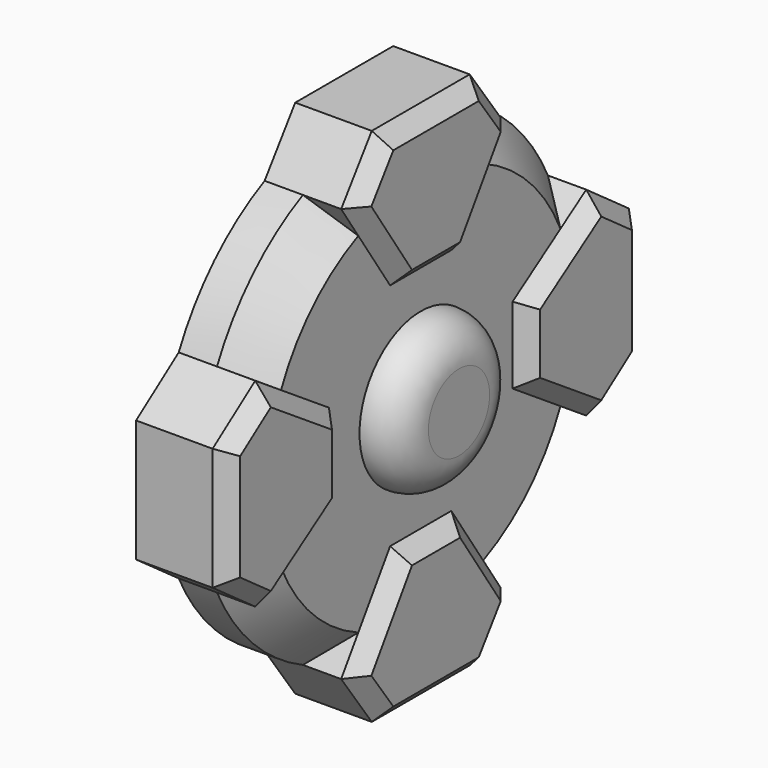
from build123d import *

# Parameters (mm, degrees)
F1_DEPTH = 10
F2_DEPTH = 12
F3_SIZE  = 5
F4_SIZE  = 1.99999
F5_R     = 10
F6_DEPTH = 5
F7_R     = 4.99999
F9_DEPTH = 9


# Not quite as in the source:
# - a fillet or chamfer is up to 0.001 mm smaller than in the source, because OpenCascade refuses the exact size


with BuildPart() as f1:
    # F0 (on Right) → F1 (new body)
    with BuildSketch(Plane.YZ):
        with BuildLine():
            Line((15, 5), (27.0370116692, 13))
            ThreePointArc((27.0370116692, 13), (21.2132034356, 21.2132034356), (13, 27.0370116692))
            Line((13, 27.0370116692), (5, 15))
            Line((5, 15), (0, 15))
            Line((0, 15), (-5, 15))
            Line((-5, 15), (-13, 27.0370116692))
            ThreePointArc((-13, 27.0370116692), (-21.2132034356, 21.2132034356), (-27.0370116692, 13))
            Line((-27.0370116692, 13), (-15, 5))
            Line((-15, 5), (-15, 0))
            Line((-15, 0), (-15, -5))
            Line((-15, -5), (-27.0370116692, -13))
            ThreePointArc((-27.0370116692, -13), (-21.2132034356, -21.2132034356), (-13, -27.0370116692))
            Line((-13, -27.0370116692), (-5, -15))
            Line((-5, -15), (0, -15))
            Line((0, -15), (5, -15))
            Line((5, -15), (13, -27.0370116692))
            ThreePointArc((13, -27.0370116692), (21.2132034356, -21.2132034356), (27.0370116692, -13))
            Line((27.0370116692, -13), (15, -5))
            Line((15, -5), (15, 0))
            Line((15, 0), (15, 5))
        make_face()
    extrude(amount=F1_DEPTH)

    # F0 (on Right) → F2 (join)
    with BuildSketch(Plane.YZ):
        with BuildLine():
            ThreePointArc((27.0370116692, -13), (29.2498747867, -6.6666952054), (30, 0))
            ThreePointArc((30, 0), (29.2498747867, 6.6666952054), (27.0370116692, 13))
            Line((27.0370116692, 13), (15, 5))
            Line((15, 5), (15, 0))
            Line((15, 0), (15, -5))
            Line((15, -5), (27.0370116692, -13))
        make_face()
        with BuildLine():
            ThreePointArc((27.0370116692, 13), (29.2498747867, 6.6666952054), (30, 0))
            ThreePointArc((30, 0), (29.2498747867, -6.6666952054), (27.0370116692, -13))
            Line((27.0370116692, -13), (34, -8))
            Line((34, -8), (34, 0))
            Line((34, 0), (34, 8))
            Line((34, 8), (27.0370116692, 13))
        make_face()
        with BuildLine():
            Line((5, 15), (13, 27.0370116692))
            ThreePointArc((13, 27.0370116692), (0, 30), (-13, 27.0370116692))
            Line((-13, 27.0370116692), (-5, 15))
            Line((-5, 15), (0, 15))
            Line((0, 15), (5, 15))
        make_face()
        with BuildLine():
            ThreePointArc((-13, 27.0370116692), (0, 30), (13, 27.0370116692))
            Line((13, 27.0370116692), (8, 34))
            Line((8, 34), (0, 34))
            Line((0, 34), (-8, 34))
            Line((-8, 34), (-13, 27.0370116692))
        make_face()
        with BuildLine():
            Line((-15, 5), (-27.0370116692, 13))
            ThreePointArc((-27.0370116692, 13), (-30, 0), (-27.0370116692, -13))
            Line((-27.0370116692, -13), (-15, -5))
            Line((-15, -5), (-15, 0))
            Line((-15, 0), (-15, 5))
        make_face()
        with BuildLine():
            ThreePointArc((-27.0370116692, -13), (-30, 0), (-27.0370116692, 13))
            Line((-27.0370116692, 13), (-34, 8))
            Line((-34, 8), (-34, 0))
            Line((-34, 0), (-34, -8))
            Line((-34, -8), (-27.0370116692, -13))
        make_face()
        with BuildLine():
            ThreePointArc((-13, -27.0370116692), (0, -30), (13, -27.0370116692))
            Line((13, -27.0370116692), (5, -15))
            Line((5, -15), (0, -15))
            Line((0, -15), (-5, -15))
            Line((-5, -15), (-13, -27.0370116692))
        make_face()
        with BuildLine():
            Line((8, -34), (13, -27.0370116692))
            ThreePointArc((13, -27.0370116692), (0, -30), (-13, -27.0370116692))
            Line((-13, -27.0370116692), (-8, -34))
            Line((-8, -34), (0, -34))
            Line((0, -34), (8, -34))
        make_face()
    extrude(amount=F2_DEPTH)

    # F3
    f3_edges = [f1.edges().sort_by_distance(p)[0] for p in [
        (10, 21.213203, 21.213203),
        (10, -21.213203, 21.213203),
        (10, -21.213203, -21.213203),
        (10, 21.213203, -21.213203),
    ]]
    chamfer(f3_edges, length=F3_SIZE)

    # F4 (size 2 in the source; OpenCascade refuses exactly that, so slightly less here)
    f4_edges = [f1.edges().sort_by_distance(p)[0] for p in [
        (12, 0, 34),
        (12, -10.5, 30.518506),
        (12, 10.5, 30.518506),
        (12, -9, 21.018506),
        (12, 9, 21.018506),
        (12, 0, 15),
        (12, -15, 0),
        (12, -21.018506, 9),
        (12, -30.518506, 10.5),
        (12, -34, 0),
        (12, -30.518506, -10.5),
        (12, -21.018506, -9),
        (12, 0, -15),
        (12, -9, -21.018506),
        (12, -10.5, -30.518506),
        (12, 0, -34),
        (12, 10.5, -30.518506),
        (12, 9, -21.018506),
        (12, 15, 0),
        (12, 21.018506, 9),
        (12, 30.518506, 10.5),
        (12, 34, 0),
        (12, 21.018506, -9),
        (12, 30.518506, -10.5),
    ]]
    chamfer(f4_edges, length=F4_SIZE)

    # F5 (on face) → F6 (join)
    with BuildSketch(Plane.YZ.offset(10)):
        Circle(F5_R)
    extrude(amount=F6_DEPTH)

    # F7 (radius 5 in the source; OpenCascade refuses exactly that, so slightly less here)
    f7_edges = [f1.edges().sort_by_distance(p)[0] for p in [
        (15, -10, 0),
    ]]
    fillet(f7_edges, radius=F7_R)

    # F8 (on face) → F9 (join)
    with BuildSketch(Plane.YZ):
        with BuildLine():
            ThreePointArc((0, -15), (10.6066017178, -10.6066017178), (15, 0))
            ThreePointArc((15, 0), (10.6066017178, 10.6066017178), (0, 15))
            ThreePointArc((0, 15), (-10.6066017178, 10.6066017178), (-15, 0))
            ThreePointArc((-15, 0), (-10.6066017178, -10.6066017178), (0, -15))
        make_face()
    extrude(amount=-F9_DEPTH)


solid = f1.part
